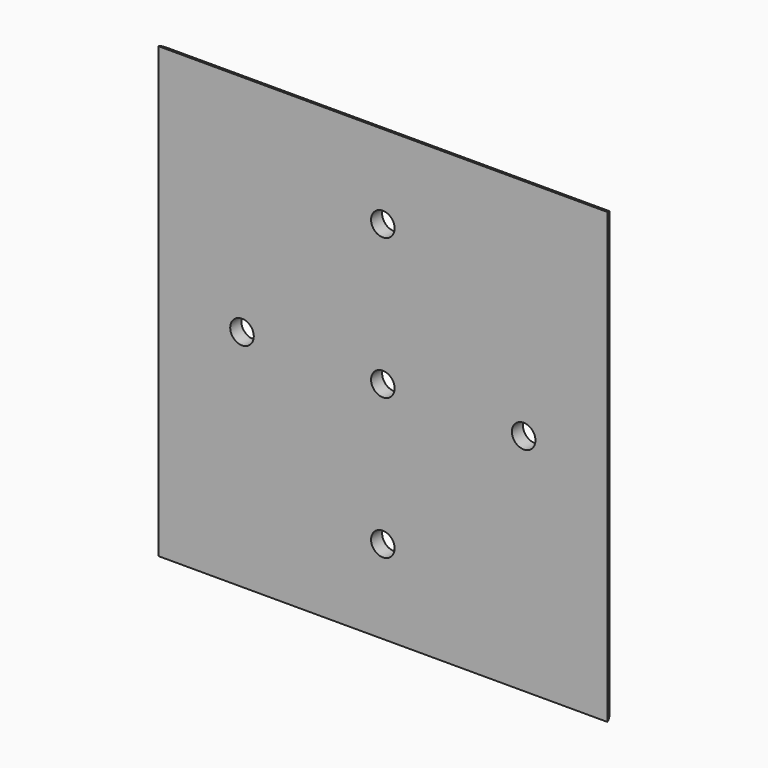
from build123d import *

# Parameters (mm, degrees)
F0_W        = 129.54
F0_H        = 129.54
F0_R        = 3.39979
F1_DEPTH    = 3.9878
F2_T1_DEPTH = 154.3459968354
F2_T3_DEPTH = 154.3459968354


# Not quite as in the source:
# - a fillet or chamfer that OpenCascade refuses, or shapes differently, is made with other operations: its cross-section is extruded or revolved along the edge and cut away or added


with BuildPart() as f1:
    # F0 (on Front) → F1 (new body)
    with BuildSketch(Plane.XZ):
        Rectangle(F0_W, F0_H)
        with Locations((0, -40.64)):
            Circle(F0_R, mode=Mode.SUBTRACT)
        with Locations((-40.64, 0)):
            Circle(F0_R, mode=Mode.SUBTRACT)
        Circle(F0_R, mode=Mode.SUBTRACT)
        with Locations((40.64, 0)):
            Circle(F0_R, mode=Mode.SUBTRACT)
        with Locations((0, 40.64)):
            Circle(F0_R, mode=Mode.SUBTRACT)
    extrude(amount=F1_DEPTH)

    # F2: fillet of radius 5.08 on 4 edges, made by hand

    # F2_s2 → F2_t1 (cut)
    with BuildSketch(Plane.XY.offset(-77.1729984177)):
        with BuildLine():
            ThreePointArc((-64.77, -3.9878), (-62.9914115108, -1.1205318539), (-59.8088006329, 0))
            Line((-59.8088006329, 0), (-64.77, 0))
            Line((-64.77, 0), (-64.77, -3.9878))
        make_face()
        with BuildLine():
            ThreePointArc((64.77, -3.9878), (62.9914115108, -1.1205318539), (59.8088006329, 0))
            Line((59.8088006329, 0), (64.77, 0))
            Line((64.77, 0), (64.77, -3.9878))
        make_face()
    extrude(amount=F2_T1_DEPTH, mode=Mode.SUBTRACT)

    # F2_s4 → F2_t3 (cut)
    with BuildSketch(Plane.YZ.offset(-77.1729984177)):
        with BuildLine():
            ThreePointArc((-3.9878, -64.77), (-1.1205318539, -62.9914115108), (0, -59.8088006329))
            Line((0, -59.8088006329), (0, -64.77))
            Line((0, -64.77), (-3.9878, -64.77))
        make_face()
        with BuildLine():
            ThreePointArc((-3.9878, 64.77), (-1.1205318539, 62.9914115108), (0, 59.8088006329))
            Line((0, 59.8088006329), (0, 64.77))
            Line((0, 64.77), (-3.9878, 64.77))
        make_face()
    extrude(amount=F2_T3_DEPTH, mode=Mode.SUBTRACT)


solid = f1.part
